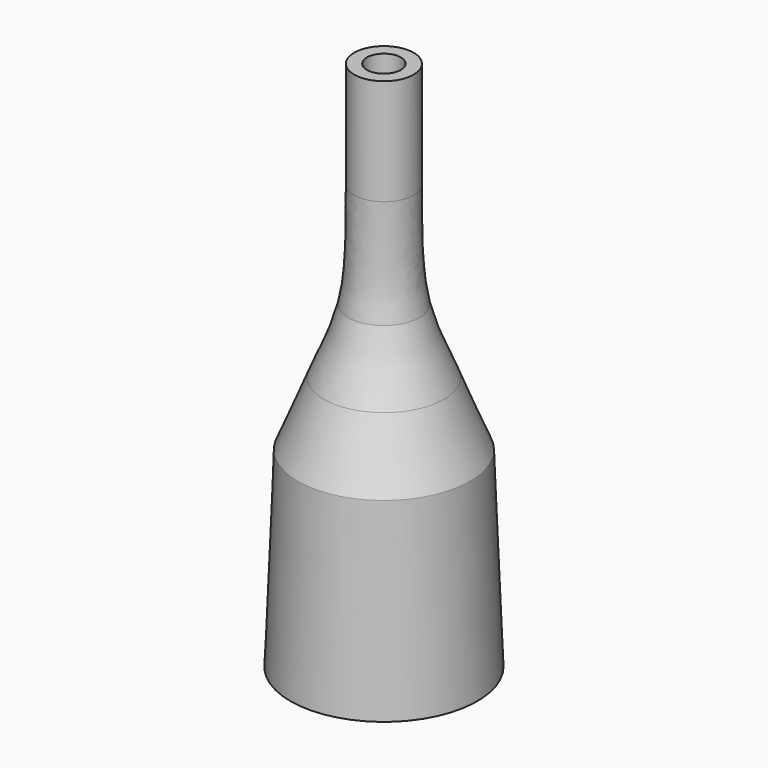
from build123d import *


with BuildPart() as f1:
    # F0 (on Front) → F1 (revolve)
    with BuildSketch(Plane.XZ):
        Polygon((-22, 0), (-17, 0), (-16.25, 45), (-20.25, 45), align=None)
    revolve(axis=Axis((0, 0, 22.5), (0, 0, 1)))

    # F0 (on Front) → F2 (revolve)
    with BuildSketch(Plane.XZ):
        with BuildLine():
            Line((-20.25, 45), (-16.25, 45))
            Line((-16.25, 45), (-10.1249999976, 59.999902775))
            add(Edge.make_bspline(
                [(-10.1249999976, 59.999902775), (-8.5298389727, 64.666048141), (-6.5813622983, 69.2951174162), (-5.4999999953, 74.9998055501)],
                knots=[0, 0, 0, 0, 0.441861733, 0.441861733, 0.441861733, 0.441861733], degree=3))
            Line((-5.4999999953, 74.9998055501), (-8.4969373337, 75.1353289405))
            add(Edge.make_bspline(
                [(-14.1249999976, 59.999902775), (-12.3183567805, 64.7249967507), (-9.8064455142, 69.3661766921), (-8.4969373337, 75.1353289405)],
                knots=[0, 0, 0, 0, 0.4460290714, 0.4460290714, 0.4460290714, 0.4460290714], degree=3))
            Line((-14.1249999976, 59.999902775), (-20.25, 45))
        make_face()
    revolve(axis=Axis((0, 0, 60), (0, 0, 1)))

    # F0 (on Front) → F3 (revolve)
    with BuildSketch(Plane.XZ):
        with BuildLine():
            Line((-8.4969373337, 75.1353289405), (-5.4999999953, 74.9998055501))
            add(Edge.make_bspline(
                [(-5.4999999953, 74.9998055501), (-4.1340756876, 82.2056903566), (-4.1516769819, 91.1277804046), (-3.9999999953, 99.9998055501)],
                knots=[0.441861733, 0.441861733, 0.441861733, 0.441861733, 1, 1, 1, 1], degree=3))
            Line((-3.9999999953, 99.9998055501), (-3.9999999953, 124.9998055501))
            Line((-3.9999999953, 124.9998055501), (-6.9999999953, 124.9998055501))
            Line((-6.9999999953, 124.9998055501), (-6.9999999953, 99.9998055501))
            add(Edge.make_bspline(
                [(-8.4969373337, 75.1353289405), (-6.8705198887, 82.3006525327), (-7.0989050536, 91.2059633256), (-6.9999999953, 99.9998055501)],
                knots=[0.4460290714, 0.4460290714, 0.4460290714, 0.4460290714, 1, 1, 1, 1], degree=3))
        make_face()
    revolve(axis=Axis((0, 0, 100), (0, 0, 1)))


solid = f1.part
